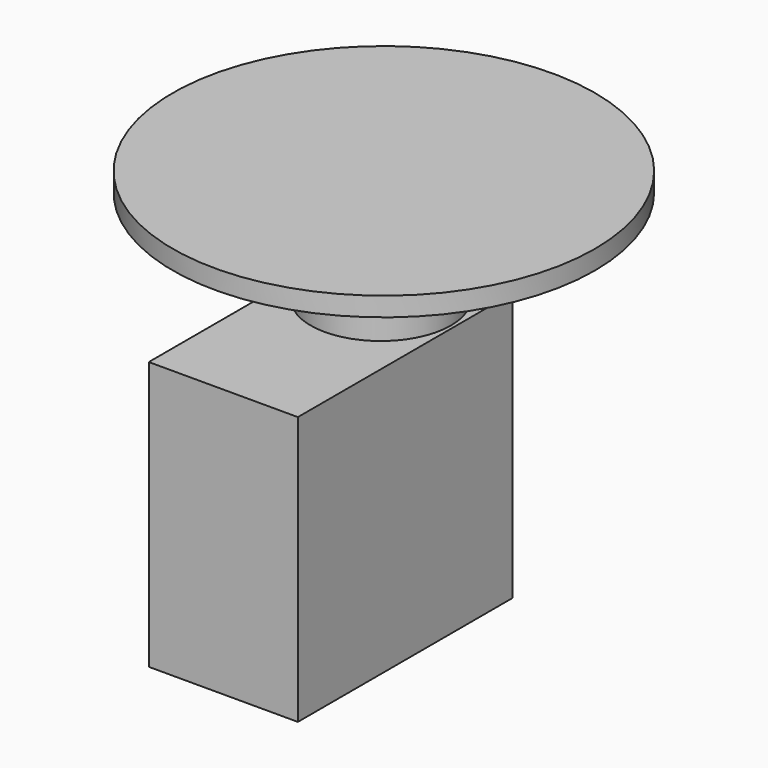
from build123d import *

# Parameters (mm, degrees)
F0_W     = 22.5
F0_H     = 22.5
F1_DEPTH = 12.5
F2_R     = 5.8842298642
F3_DEPTH = 26.6
F6_R     = 17.7
F7_DEPTH = 1.6


# Not quite as in the source:
# - the program builds the solid bodies; features that only make, move or delete a surface that nothing else refers to are left out


with BuildPart() as f1:
    # F0 (on Right) → F1 (new body)
    with BuildSketch(Plane.YZ):
        with Locations((11.25, 11.25)):
            Rectangle(F0_W, F0_H)
    extrude(amount=F1_DEPTH)

    # F2 (on Top) → F3 (join)
    with BuildSketch(Plane.XY):
        with Locations((6.3317283057, 16.4049286395)):
            Circle(F2_R)
    extrude(amount=F3_DEPTH)


with BuildPart() as f7:
    # F6 (on Top) → F7 (new body)
    with BuildSketch(Plane.XY):
        with Locations((61.9552992284, -52.9340319335)):
            Circle(F6_R)
    extrude(amount=F7_DEPTH)


with BuildPart() as f8_1:
    # F8: copy of F7
    add(f7.part.moved(Location((-55.372, 69.342, 30.48))))


solid = Compound([f1.part, f8_1.part])
